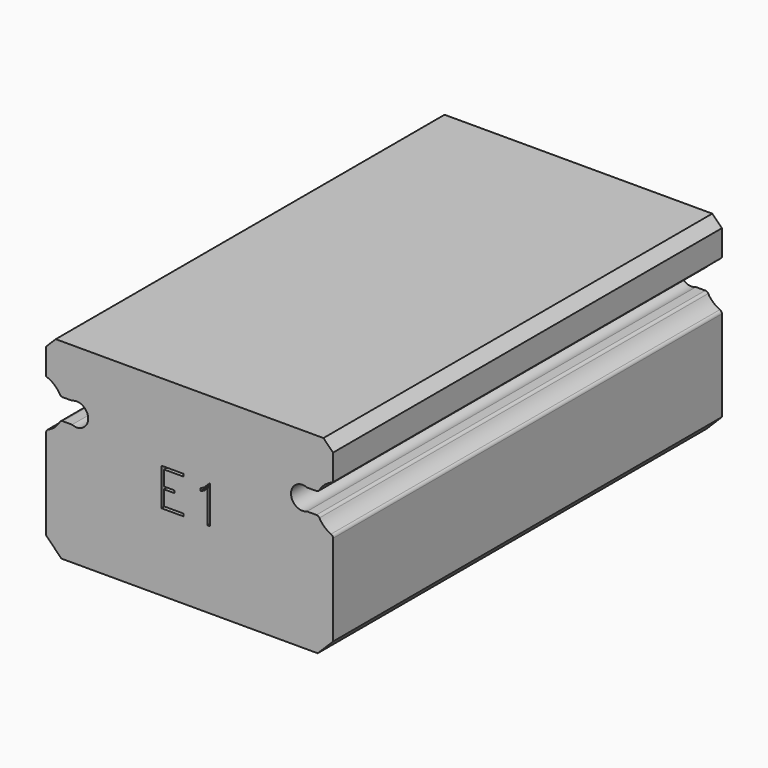
from build123d import *

# Parameters (mm, degrees)
F1_DEPTH = 25.4


# Not quite as in the source:
# - ends of sketch curves that miss each other by under 0.0002 mm in the source are joined


with BuildPart() as f1:
    # F0 (on Front) → F1 (new body)
    with BuildSketch(Plane.XZ):
        with BuildLine():
            Line((-7.5, -7.195485), (-6.695486, -8))
            Line((-6.695486, -8), (6.695486, -8))
            Line((6.695486, -8), (7.5, -7.195485))
            Line((7.5, -7.195485), (7.5, -2.445548))
            ThreePointArc((7.5, -2.445548), (7.4679364252, -2.3523462741), (7.3915955611, -2.2900030169))
            ThreePointArc((7.3915955611, -2.2900030169), (7.0435250993, -2.0677653184), (6.7835181408, -1.7469249193))
            ThreePointArc((6.7835181408, -1.7469249193), (6.7175952727, -1.6806726709), (6.627337, -1.656408))
            Line((6.627337, -1.656408), (6.138893, -1.656409))
            ThreePointArc((6.138893, -1.656409), (5.300907, -1.105625), (6.1388920414, -0.5548409043))
            Line((6.1388920414, -0.5548409043), (6.627337, -0.554841))
            ThreePointArc((6.627337, -0.554841), (6.7175947713, -0.5305764639), (6.7835185098, -0.4643247191))
            ThreePointArc((6.7835185098, -0.4643247191), (7.0715565387, -0.1191653097), (7.4605499849, 0.1061910414))
            ThreePointArc((7.4605499849, 0.1061910414), (7.4891585913, 0.1281728571), (7.5, 0.162584))
            Line((7.5, 0.162584), (7.5, 1.495485))
            Line((7.5, 1.495485), (6.995485, 2))
            Line((6.995485, 2), (-6.995485, 2))
            Line((-6.995485, 2), (-7.5, 1.495485))
            Line((-7.5, 1.495485), (-7.5, 0.162584))
            ThreePointArc((-7.5, 0.162584), (-7.489158493, 0.1281727166), (-7.460549826, 0.1061904768))
            ThreePointArc((-7.460549826, 0.1061904768), (-7.0715565387, -0.1191653097), (-6.7835181408, -0.4643250807))
            ThreePointArc((-6.7835181408, -0.4643250807), (-6.7175952727, -0.5305773291), (-6.627337, -0.554842))
            Line((-6.627337, -0.554842), (-6.138893, -0.554841))
            ThreePointArc((-6.138893, -0.554841), (-5.300907, -1.105625), (-6.1388920414, -1.6564090957))
            Line((-6.1388920414, -1.6564090957), (-6.627337, -1.656409))
            ThreePointArc((-6.627337, -1.656409), (-6.7175947713, -1.6806735361), (-6.7835185098, -1.7469252809))
            ThreePointArc((-6.7835185098, -1.7469252809), (-7.0435250993, -2.0677653184), (-7.3915951882, -2.290002564))
            ThreePointArc((-7.3915951882, -2.290002564), (-7.467936276, -2.35234606), (-7.499999532, -2.4455480253))
            Line((-7.499999532, -2.4455480253), (-7.5, -7.195485))
        make_face()
        Polygon((-0.330203, -3.983), (-1.467667, -3.983), (-1.467667, -2.023), (-0.330203, -2.023), (-0.330203, -2.153666), (-1.337, -2.153666), (-1.337, -2.937667), (-0.788302, -2.937667), (-0.788302, -3.068333), (-1.337, -3.068333), (-1.337, -3.852334), (-0.330203, -3.852334), align=None, mode=Mode.SUBTRACT)
        Polygon((1.064667, -3.985533), (0.934, -3.985533), (0.934, -2.278991), (0.784703, -2.429492), (0.567776, -2.536533), (0.567776, -2.398867), (0.759182, -2.302033), (1.037104, -2.025533), (1.064667, -2.025533), align=None, mode=Mode.SUBTRACT)
    extrude(amount=F1_DEPTH)


solid = f1.part
